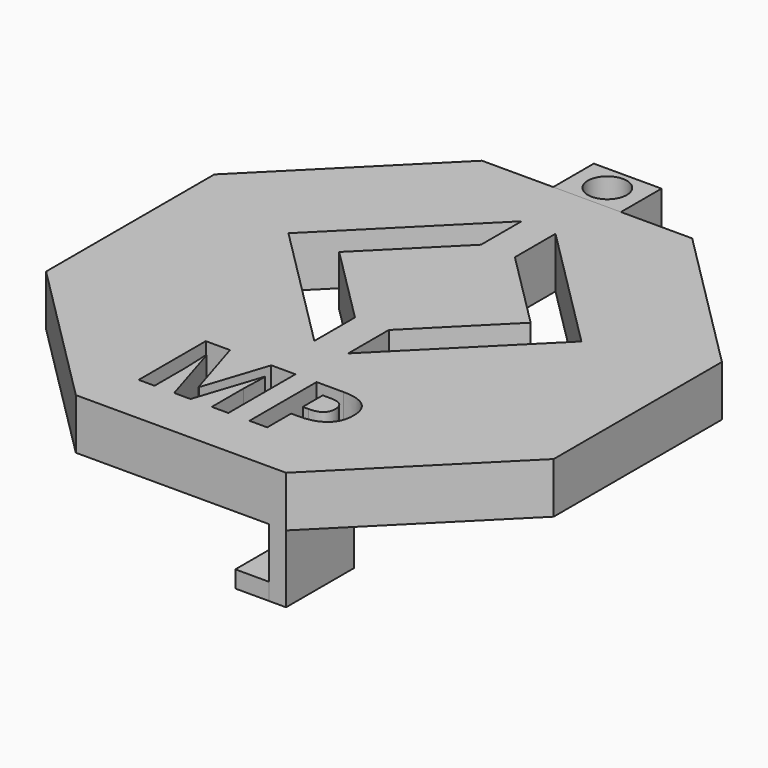
from build123d import *

# Parameters (mm, degrees)
F1_DEPTH     = 3
F2_TEXT_SIZE = 6.9444444444
F3_DEPTH     = 3.001
F4_W         = 1
F4_H         = 5
F5_DEPTH     = 4
F6_W         = 5
F6_H         = 1
F7_DEPTH     = 2
F8_W         = 4
F8_H         = 3
F9_DEPTH     = 3
F10_R        = 1.15
F11_DEPTH    = 3.0010001


# Not quite as in the source:
# - Text() gives the source's letters only with a copy of the font that has no kerning and outlines rounded to 1/6400 em; it was checked with that copy


with BuildPart() as f1:
    # F0 (on Top) → F1 (new body)
    with BuildSketch(Plane.XY):
        Polygon((15, -6.2132034356), (15, 6.2132034356), (6.2132034356, 15), (-6.2132034356, 15), (-15, 6.2132034356), (-15, -6.2132034356), (-6.2132034356, -15), (6.2132034356, -15), align=None)
    extrude(amount=F1_DEPTH)

    # F2 (on face) → F3 (cut, through all)
    with BuildSketch(Plane.XY.offset(3)):
        Polygon((1, 8.418436326), (5.6568542495, 3.7615820765), (1, -0.8952721729), (1, -3.8952721729), (8.6568542495, 3.7615820765), (1, 11.418436326), align=None)
        Polygon((-1, -0.8952721729), (-5.6568542495, 3.7615820765), (-1, 8.418436326), (-1, 11.418436326), (-8.6568542495, 3.7615820765), (-1, -3.8952721729), align=None)
        with Locations((-5.5230034722, -12)):
            Text('MP', F2_TEXT_SIZE, font='Open Sans', font_style=FontStyle.BOLD, text_align=(TextAlign.LEFT, TextAlign.BOTTOM))
    extrude(amount=-F3_DEPTH, mode=Mode.SUBTRACT)

    # F4 (on face) → F5 (join)
    with BuildSketch(Plane(origin=(0, 0, 0), x_dir=(1, 0, 0), z_dir=(0, 0, -1))):
        with Locations((5.7132034356, 12.5)):
            Rectangle(F4_W, F4_H)
    extrude(amount=F5_DEPTH)


with BuildPart() as f7:
    # F6 (on face) → F7 (new body)
    with BuildSketch(Plane(origin=(5.2132034356, 0, 0), x_dir=(0, -1, 0), z_dir=(-1, 0, 0))):
        with Locations((12.5, -3.5)):
            Rectangle(F6_W, F6_H)
    extrude(amount=F7_DEPTH)


with BuildPart() as f9:
    # F8 (on face) → F9 (new body)
    with BuildSketch(Plane(origin=(0, 15, 0), x_dir=(-1, 0, 0), z_dir=(0, 1, 0))):
        with Locations((0, 1.5)):
            Rectangle(F8_W, F8_H)
    extrude(amount=F9_DEPTH)

    # F10 (on face) → F11 (cut, through all)
    with BuildSketch(Plane(origin=(0, 0, 0), x_dir=(1, 0, 0), z_dir=(0, 0, -1))):
        with Locations((0, -16.5)):
            Circle(F10_R)
    extrude(amount=-F11_DEPTH, mode=Mode.SUBTRACT)


solid = Compound([f1.part, f7.part, f9.part])
